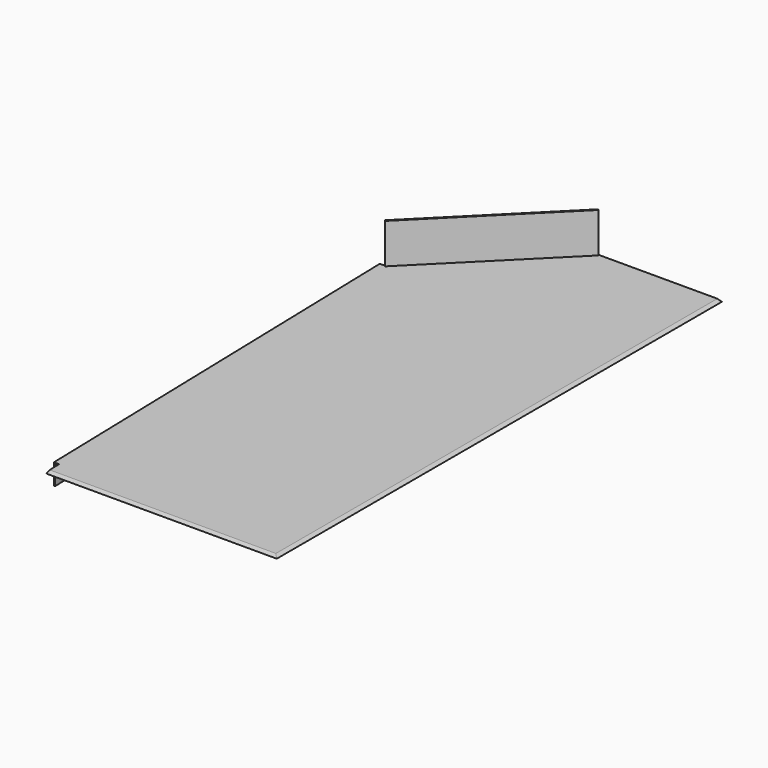
from build123d import *

# Parameters (mm, degrees)
F2_DEPTH  = 1.524
F3_W      = 519.1125
F3_H      = 25.4
F4_DEPTH  = 1.524
F6_DEPTH  = 50.8
F8_DEPTH  = 685.801
F10_DEPTH = 304.801


# Not quite as in the source:
# - a variable given as a bare number and used for a length is read in inches; the dataset says mm whatever the document's units were


with BuildPart() as f2:
    # F1 (on Top) → F2 (new body)
    with BuildSketch(Plane.XY):
        Polygon((0, 0), (-152.4021759864, 0), (-298.4521759864, -146.05), (-304.8, -146.2162236218), (-291.2112189215, -665.1508367331), (-284.8633949079, -664.9846131114), (-284.3183248194, -685.8), (0, -685.8), align=None)
    extrude(amount=F2_DEPTH)

    # F3 (on face) → F4 (join)
    with BuildSketch(Plane(origin=(-308.4173240373, -8.0761918578, 0), x_dir=(0.0261769483, -0.999657325, 0), z_dir=(-0.999657325, -0.0261769483, 0))):
        with Locations((397.7436351295, -11.176)):
            Rectangle(F3_W, F3_H)
    extrude(amount=-F4_DEPTH)

    # F5 (on Top) → F6 (join)
    with BuildSketch(Plane.XY):
        Polygon((-152.4021759864, 0), (-298.4521759864, -146.05), (-297.3745452519, -147.1276307345), (-151.3245452519, -1.0776307345), align=None)
    extrude(amount=F6_DEPTH)

    # F7 (on Front) → F8 (cut, through all)
    with BuildSketch(Plane.XZ):
        Polygon((6.35, 4.6485226281), (-17.3485226281, 4.6485226281), (6.35, -1.7014773719), align=None)
    extrude(amount=F8_DEPTH, mode=Mode.SUBTRACT)

    # F9 (on Right) → F10 (cut, through all)
    with BuildSketch(Plane.YZ):
        Polygon((-668.4514773719, 4.6485226281), (-692.15, 4.6485226281), (-692.15, -1.7014773719), align=None)
    extrude(amount=-F10_DEPTH, mode=Mode.SUBTRACT)


solid = f2.part
